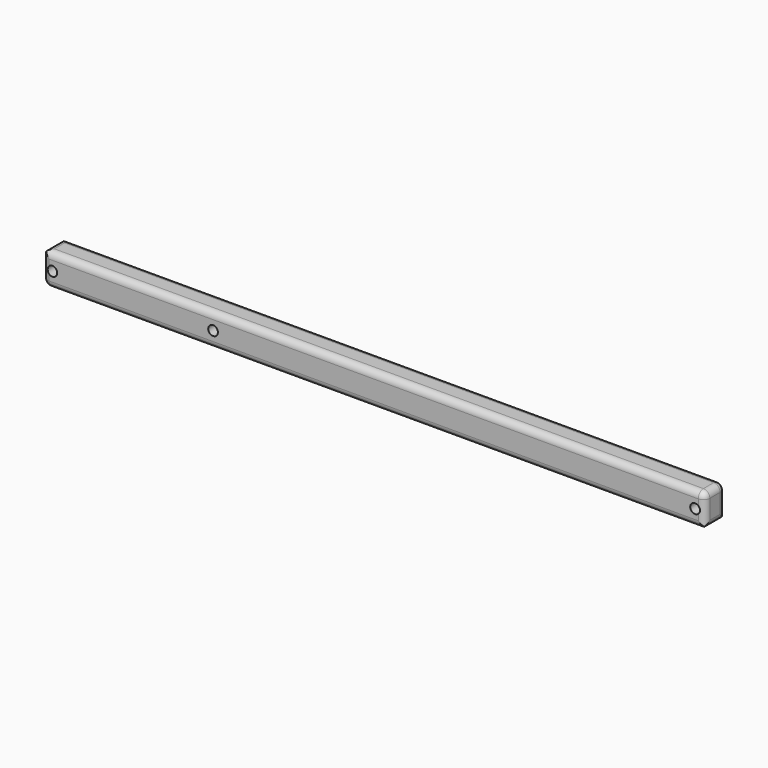
from build123d import *

# Parameters (mm, degrees)
F0_W         = 206
F0_H         = 10
F0_R         = 1.5
F1_DEPTH     = 8
F2_T1_DEPTH  = 4
F2_T3_DEPTH  = 18
F2_T5_DEPTH  = 209
F2_T7_DEPTH  = 13
F2_S11_W     = 2
F2_S11_H     = 2
F2_T12_DEPTH = 2
F2_S17_W     = 2
F2_S17_H     = 2
F2_T18_DEPTH = 2
F3_T1_DEPTH  = 11
F3_T3_DEPTH  = 4
F3_T5_DEPTH  = 207
F3_S9_W      = 2.04
F3_S9_H      = 2.04
F3_T10_DEPTH = 2.04
F3_S15_W     = 2.04
F3_S15_H     = 2.04
F3_T16_DEPTH = 2.04


# Not quite as in the source:
# - a fillet or chamfer that OpenCascade refuses, or shapes differently, is made with other operations: its cross-section is extruded or revolved along the edge and cut away or added


with BuildPart() as f1:
    # F0 (on Front) → F1 (new body)
    with BuildSketch(Plane.XZ):
        with Locations((-40, 5)):
            Rectangle(F0_W, F0_H)
        with Locations((-140, 5)):
            Circle(F0_R, mode=Mode.SUBTRACT)
        with Locations((-90, 5)):
            Circle(F0_R, mode=Mode.SUBTRACT)
        with Locations((60, 5)):
            Circle(F0_R, mode=Mode.SUBTRACT)
    extrude(amount=F1_DEPTH)

    # F2: fillet of radius 2 on 7 edges, made by hand

    # F2_s2 → F2_t1 (cut)
    with BuildSketch(Plane.XZ.offset(2)):
        with BuildLine():
            ThreePointArc((63, 8), (62.4142135624, 9.4142135624), (61, 10))
            Line((61, 10), (63, 10))
            Line((63, 10), (63, 8))
        make_face()
    extrude(amount=F2_T1_DEPTH, mode=Mode.SUBTRACT)

    # F2_s4 → F2_t3 (cut)
    with BuildSketch(Plane.XZ.offset(-5)):
        with BuildLine():
            ThreePointArc((-143, 8), (-142.4142135624, 9.4142135624), (-141, 10))
            Line((-141, 10), (-143, 10))
            Line((-143, 10), (-143, 8))
        make_face()
        with BuildLine():
            ThreePointArc((61, 0), (62.4142135624, 0.5857864376), (63, 2))
            Line((63, 2), (63, 0))
            Line((63, 0), (61, 0))
        make_face()
    extrude(amount=F2_T3_DEPTH, mode=Mode.SUBTRACT)

    # F2_s6 → F2_t5 (cut)
    with BuildSketch(Plane.YZ.offset(-148)):
        with BuildLine():
            ThreePointArc((-2, 10), (-0.5857864376, 9.4142135624), (0, 8))
            Line((0, 8), (0, 10))
            Line((0, 10), (-2, 10))
        make_face()
        with BuildLine():
            ThreePointArc((-6, 10), (-7.4142135624, 9.4142135624), (-8, 8))
            Line((-8, 8), (-8, 10))
            Line((-8, 10), (-6, 10))
        make_face()
    extrude(amount=F2_T5_DEPTH, mode=Mode.SUBTRACT)

    # F2_s8 → F2_t7 (cut)
    with BuildSketch(Plane.XY.offset(-5)):
        with BuildLine():
            ThreePointArc((63, -2), (62.4142135624, -0.5857864376), (61, 0))
            Line((61, 0), (63, 0))
            Line((63, 0), (63, -2))
        make_face()
        with BuildLine():
            ThreePointArc((63, -6), (62.4142135624, -7.4142135624), (61, -8))
            Line((61, -8), (63, -8))
            Line((63, -8), (63, -6))
        make_face()
    extrude(amount=F2_T7_DEPTH, mode=Mode.SUBTRACT)


with BuildPart() as f2_tool10:
    # F2_s11 → F2_t12 (new body)
    with BuildSketch(Plane.YZ.offset(61)):
        with Locations((-1, 9)):
            Rectangle(F2_S11_W, F2_S11_H)
    extrude(amount=F2_T12_DEPTH)

    # F2_s13 → F2_t14 (revolve, cut)
    with BuildSketch(Plane(origin=(61, -2, 8), x_dir=(0, -0.7071067812, -0.7071067812), z_dir=(0, -0.7071067812, 0.7071067812))):
        with BuildLine():
            ThreePointArc((0, -2), (2, 0), (0, 2))
            Line((0, 2), (0, -2))
        make_face()
    revolve(axis=Axis((61, -2, 8), (1, 0, 0)), mode=Mode.SUBTRACT)


with BuildPart() as f1_1:
    add(f1.part)

    # F2_t9: cut F2_tool10
    add(f2_tool10.part, mode=Mode.SUBTRACT)


with BuildPart() as f2_tool16:
    # F2_s17 → F2_t18 (new body)
    with BuildSketch(Plane.XZ.offset(6)):
        with Locations((62, 9)):
            Rectangle(F2_S17_W, F2_S17_H)
    extrude(amount=F2_T18_DEPTH)

    # F2_s19 → F2_t20 (revolve, cut)
    with BuildSketch(Plane(origin=(61, -6, 8), x_dir=(-0.7071067812, 0, -0.7071067812), z_dir=(-0.7071067812, 0, 0.7071067812))):
        with BuildLine():
            ThreePointArc((0, -2), (2, 0), (0, 2))
            Line((0, 2), (0, -2))
        make_face()
    revolve(axis=Axis((61, -6, 8), (0, -1, 0)), mode=Mode.SUBTRACT)


with BuildPart() as f1_2:
    add(f1_1.part)

    # F2_t15: cut F2_tool16
    add(f2_tool16.part, mode=Mode.SUBTRACT)

    # F3: fillet of radius 2 on 7 edges, made by hand

    # F3_s2 → F3_t1 (cut)
    with BuildSketch(Plane.XY.offset(2)):
        with BuildLine():
            ThreePointArc((-143, -2), (-142.4142135624, -0.5857864376), (-141, 0))
            Line((-141, 0), (-143, 0))
            Line((-143, 0), (-143, -2))
        make_face()
        with BuildLine():
            ThreePointArc((-143, -6), (-142.4142135624, -7.4142135624), (-141, -8))
            Line((-141, -8), (-143, -8))
            Line((-143, -8), (-143, -6))
        make_face()
    extrude(amount=F3_T1_DEPTH, mode=Mode.SUBTRACT)

    # F3_s4 → F3_t3 (cut)
    with BuildSketch(Plane.XZ.offset(2)):
        with BuildLine():
            ThreePointArc((-143, 2), (-142.4142135624, 0.5857864376), (-141, 0))
            Line((-141, 0), (-143, 0))
            Line((-143, 0), (-143, 2))
        make_face()
    extrude(amount=F3_T3_DEPTH, mode=Mode.SUBTRACT)

    # F3_s6 → F3_t5 (cut)
    with BuildSketch(Plane.YZ.offset(-141)):
        with BuildLine():
            ThreePointArc((0, 2), (-0.5857864376, 0.5857864376), (-2, 0))
            Line((-2, 0), (0, 0))
            Line((0, 0), (0, 2))
        make_face()
        with BuildLine():
            ThreePointArc((-6, 0), (-7.4142135624, 0.5857864376), (-8, 2))
            Line((-8, 2), (-8, 0))
            Line((-8, 0), (-6, 0))
        make_face()
    extrude(amount=F3_T5_DEPTH, mode=Mode.SUBTRACT)


with BuildPart() as f3_tool8:
    # F3_s9 → F3_t10 (new body)
    with BuildSketch(Plane.YZ.offset(-141)):
        with Locations((-0.98, 0.98)):
            Rectangle(F3_S9_W, F3_S9_H)
    extrude(amount=-F3_T10_DEPTH)

    # F3_s11 → F3_t12 (revolve, cut)
    with BuildSketch(Plane(origin=(-141, -2, 2), x_dir=(0, -0.7071067812, 0.7071067812), z_dir=(0, -0.7071067812, -0.7071067812))):
        with BuildLine():
            ThreePointArc((0, -2), (2, 0), (0, 2))
            Line((0, 2), (0, -2))
        make_face()
    revolve(axis=Axis((-141, -2, 2), (-1, 0, 0)), mode=Mode.SUBTRACT)


with BuildPart() as f1_3:
    add(f1_2.part)

    # F3_t7: cut F3_tool8
    add(f3_tool8.part, mode=Mode.SUBTRACT)


with BuildPart() as f3_tool14:
    # F3_s15 → F3_t16 (new body)
    with BuildSketch(Plane.YZ.offset(-141)):
        with Locations((-7.02, 0.98)):
            Rectangle(F3_S15_W, F3_S15_H)
    extrude(amount=-F3_T16_DEPTH)

    # F3_s17 → F3_t18 (revolve, cut)
    with BuildSketch(Plane(origin=(-141, -6, 2), x_dir=(0, 0.7071067812, 0.7071067812), z_dir=(0, -0.7071067812, 0.7071067812))):
        with BuildLine():
            ThreePointArc((0, -2), (2, 0), (0, 2))
            Line((0, 2), (0, -2))
        make_face()
    revolve(axis=Axis((-141, -6, 2), (-1, 0, 0)), mode=Mode.SUBTRACT)


with BuildPart() as f1_4:
    add(f1_3.part)

    # F3_t13: cut F3_tool14
    add(f3_tool14.part, mode=Mode.SUBTRACT)


solid = f1_4.part
